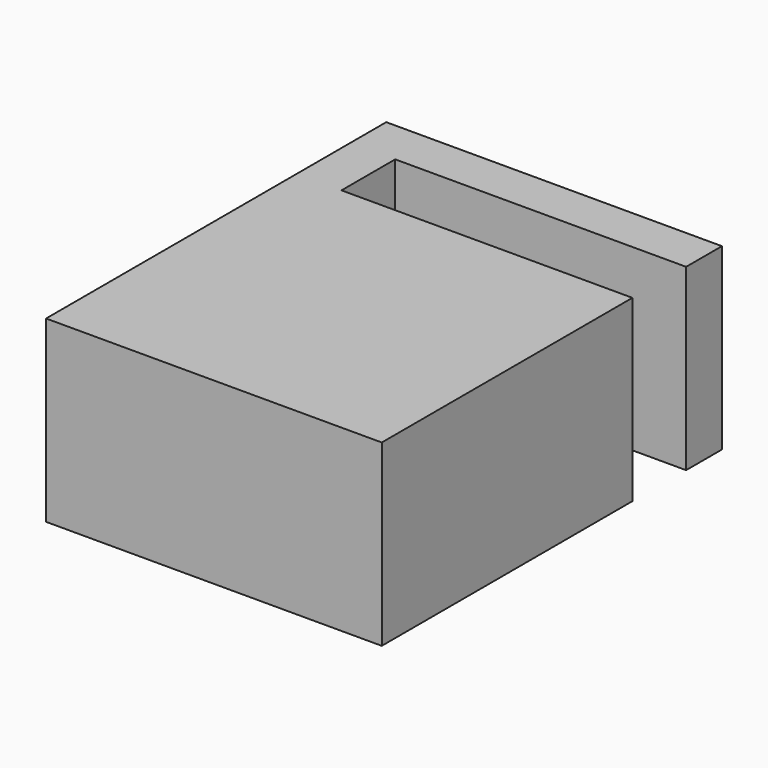
from build123d import *

# Parameters (mm, degrees)
F1_DEPTH = 8
F2_R     = 1.7
F3_DEPTH = 0.5
F4_R     = 0.49999


# Not quite as in the source:
# - a fillet or chamfer is up to 0.001 mm smaller than in the source, because OpenCascade refuses the exact size


with BuildPart() as f1:
    # F0 (on Top) → F1 (new body)
    with BuildSketch(Plane.XY):
        Polygon((-7.5, -9.5), (7.5, -9.5), (7.5, 4.5), (-5.5, 4.5), (-5.5, 7.5), (7.5, 7.5), (7.5, 9.5), (-7.5, 9.5), align=None)
    extrude(amount=F1_DEPTH)

    # F2 (on face) → F3 (join)
    with BuildSketch(Plane.XZ.offset(-7.5)):
        with Locations((2, 4)):
            Circle(F2_R)
    extrude(amount=F3_DEPTH)

    # F4 (radius 0.5 in the source; OpenCascade refuses exactly that, so slightly less here)
    f4_edges = [f1.edges().sort_by_distance(p)[0] for p in [
        (0.3, 7, 4),
    ]]
    fillet(f4_edges, radius=F4_R)


solid = f1.part
